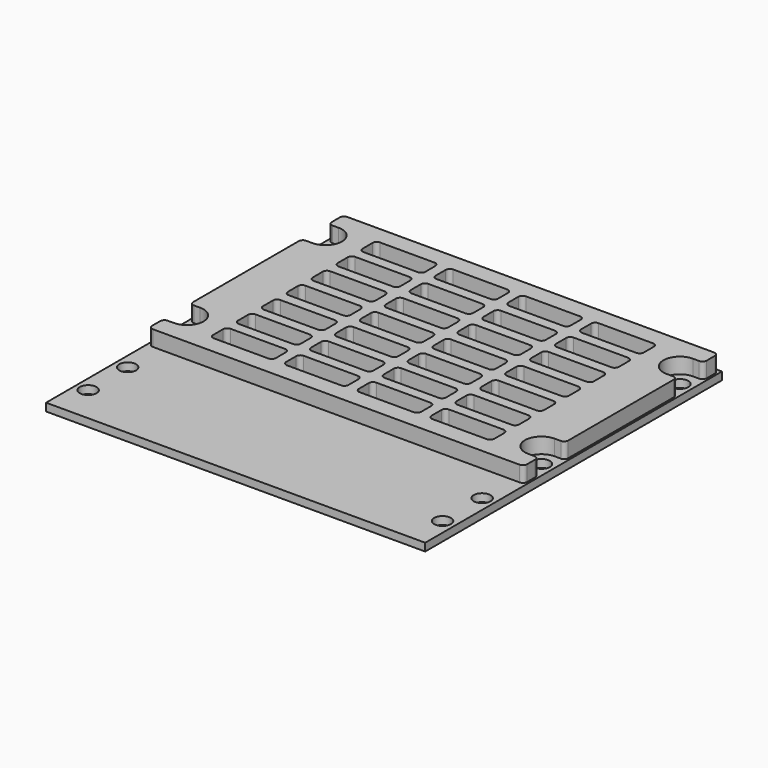
from build123d import *

# Parameters (mm, degrees)
F0_R      = 3.24
F1_DEPTH  = 3
F2_DEPTH  = 6
F3_R      = 1.588
F4_W      = 24
F4_H      = 8
F4_W_2    = 24.1504099965
F5_DEPTH  = 25
F6_R      = 1.588
F6_2_R    = 1.588
F7_W      = 108.300819993
F7_H      = 80
F8_DEPTH  = 25
F9_R      = 3.24
F10_DEPTH = 3


# Not quite as in the source:
# - a feature names something its author has since deleted; it is built from what else it names


with BuildPart() as f1:
    # F0 (on Top) → F1 (new body)
    with BuildSketch(Plane.XY):
        Polygon((0, 57.15), (-73.025, 57.15), (-73.025, 9.525), (-73.025, -38.1), (73.025, -38.1), (73.025, 57.15), align=None)
        with Locations((-68.262, -23.812)):
            Circle(F0_R, mode=Mode.SUBTRACT)
        with Locations((68.262, -23.812)):
            Circle(F0_R, mode=Mode.SUBTRACT)
        with Locations((-68.262, 42.862)):
            Circle(F0_R, mode=Mode.SUBTRACT)
        with BuildLine():
            Line((-72.225, -17.461), (-72.225, 9.525))
            Line((-72.225, 9.525), (-72.225, 36.511))
            Line((-72.225, 36.511), (-68.262, 36.511))
            ThreePointArc((-68.262, 36.511), (-61.911, 42.862), (-68.262, 49.213))
            Line((-68.262, 49.213), (-72.225, 49.213))
            Line((-72.225, 49.213), (-72.225, 56.35))
            Line((-72.225, 56.35), (72.225, 56.35))
            Line((72.225, 56.35), (72.225, 49.213))
            Line((72.225, 49.213), (68.262, 49.213))
            ThreePointArc((68.262, 49.213), (61.911, 42.862), (68.262, 36.511))
            Line((68.262, 36.511), (72.225, 36.511))
            Line((72.225, 36.511), (72.225, -17.461))
            Line((72.225, -17.461), (68.262, -17.461))
            ThreePointArc((68.262, -17.461), (61.911, -23.812), (68.262, -30.163))
            Line((68.262, -30.163), (72.225, -30.163))
            Line((72.225, -30.163), (72.225, -37.3))
            Line((72.225, -37.3), (-72.225, -37.3))
            Line((-72.225, -37.3), (-72.225, -30.163))
            Line((-72.225, -30.163), (-68.262, -30.163))
            ThreePointArc((-68.262, -30.163), (-61.911, -23.812), (-68.262, -17.461))
            Line((-68.262, -17.461), (-72.225, -17.461))
        make_face(mode=Mode.SUBTRACT)
        with Locations((68.262, 42.862)):
            Circle(F0_R, mode=Mode.SUBTRACT)
        with BuildLine():
            Line((-72.225, 36.511), (-72.225, 9.525))
            Line((-72.225, 9.525), (-72.225, -17.461))
            Line((-72.225, -17.461), (-68.262, -17.461))
            ThreePointArc((-68.262, -17.461), (-61.911, -23.812), (-68.262, -30.163))
            Line((-68.262, -30.163), (-72.225, -30.163))
            Line((-72.225, -30.163), (-72.225, -37.3))
            Line((-72.225, -37.3), (72.225, -37.3))
            Line((72.225, -37.3), (72.225, -30.163))
            Line((72.225, -30.163), (68.262, -30.163))
            ThreePointArc((68.262, -30.163), (61.911, -23.812), (68.262, -17.461))
            Line((68.262, -17.461), (72.225, -17.461))
            Line((72.225, -17.461), (72.225, 36.511))
            Line((72.225, 36.511), (68.262, 36.511))
            ThreePointArc((68.262, 36.511), (61.911, 42.862), (68.262, 49.213))
            Line((68.262, 49.213), (72.225, 49.213))
            Line((72.225, 49.213), (72.225, 56.35))
            Line((72.225, 56.35), (-72.225, 56.35))
            Line((-72.225, 56.35), (-72.225, 49.213))
            Line((-72.225, 49.213), (-68.262, 49.213))
            ThreePointArc((-68.262, 49.213), (-61.911, 42.862), (-68.262, 36.511))
            Line((-68.262, 36.511), (-72.225, 36.511))
        make_face()
    extrude(amount=-F1_DEPTH)


with BuildPart() as f2:
    # F0 (on Top) → F2 (new body)
    with BuildSketch(Plane.XY):
        with BuildLine():
            Line((-72.225, 36.511), (-72.225, 9.525))
            Line((-72.225, 9.525), (-72.225, -17.461))
            Line((-72.225, -17.461), (-68.262, -17.461))
            ThreePointArc((-68.262, -17.461), (-61.911, -23.812), (-68.262, -30.163))
            Line((-68.262, -30.163), (-72.225, -30.163))
            Line((-72.225, -30.163), (-72.225, -37.3))
            Line((-72.225, -37.3), (72.225, -37.3))
            Line((72.225, -37.3), (72.225, -30.163))
            Line((72.225, -30.163), (68.262, -30.163))
            ThreePointArc((68.262, -30.163), (61.911, -23.812), (68.262, -17.461))
            Line((68.262, -17.461), (72.225, -17.461))
            Line((72.225, -17.461), (72.225, 36.511))
            Line((72.225, 36.511), (68.262, 36.511))
            ThreePointArc((68.262, 36.511), (61.911, 42.862), (68.262, 49.213))
            Line((68.262, 49.213), (72.225, 49.213))
            Line((72.225, 49.213), (72.225, 56.35))
            Line((72.225, 56.35), (-72.225, 56.35))
            Line((-72.225, 56.35), (-72.225, 49.213))
            Line((-72.225, 49.213), (-68.262, 49.213))
            ThreePointArc((-68.262, 49.213), (-61.911, 42.862), (-68.262, 36.511))
            Line((-68.262, 36.511), (-72.225, 36.511))
        make_face()
    extrude(amount=F2_DEPTH)

    # F3
    f3_edges = [f2.edges().sort_by_distance(p)[0] for p in [
        (-72.225, 56.35, 3),
        (-72.225, -37.3, 3),
        (72.225, -37.3, 3),
        (72.225, 56.35, 3),
        (-72.225, 36.511, 3),
        (-72.225, -17.461, 3),
        (-72.225, 49.213, 3),
        (72.225, 49.213, 3),
        (72.225, 36.511, 3),
        (72.225, -17.461, 3),
        (72.225, -30.163, 3),
        (-72.225, -30.163, 3),
    ]]
    fillet(f3_edges, radius=F3_R)


with BuildPart() as f5_tool:
    # F4 (on face) → F5 (new body)
    with BuildSketch(Plane.XY.offset(6)):
        with Locations((-14, 45.525)):
            Rectangle(F4_W, F4_H)
        with Locations((-42.0752049983, 45.525)):
            Rectangle(F4_W_2, F4_H)
        with Locations((42.0752049983, 45.525)):
            Rectangle(F4_W_2, F4_H)
        with Locations((14, 45.525)):
            Rectangle(F4_W, F4_H)
        with Locations((-14, 33.525)):
            Rectangle(F4_W, F4_H)
        with Locations((-42.0752049983, 33.525)):
            Rectangle(F4_W_2, F4_H)
        with Locations((14, 33.525)):
            Rectangle(F4_W, F4_H)
        with Locations((42.0752049983, 33.525)):
            Rectangle(F4_W_2, F4_H)
        with Locations((-14, 21.525)):
            Rectangle(F4_W, F4_H)
        with Locations((-42.0752049983, 21.525)):
            Rectangle(F4_W_2, F4_H)
        with Locations((14, 21.525)):
            Rectangle(F4_W, F4_H)
        with Locations((42.0752049983, 21.525)):
            Rectangle(F4_W_2, F4_H)
        Polygon((-2, 9.525), (-2, 13.525), (-26, 13.525), (-26, 5.525), (-2, 5.525), align=None)
        with Locations((-42.0752049983, 9.525)):
            Rectangle(F4_W_2, F4_H)
        with Locations((14, 9.525)):
            Rectangle(F4_W, F4_H)
        with Locations((42.0752049983, 9.525)):
            Rectangle(F4_W_2, F4_H)
        with Locations((-14, -2.475)):
            Rectangle(F4_W, F4_H)
        with Locations((-42.0752049983, -2.475)):
            Rectangle(F4_W_2, F4_H)
        with Locations((14, -2.475)):
            Rectangle(F4_W, F4_H)
        with Locations((42.0752049983, -2.475)):
            Rectangle(F4_W_2, F4_H)
        with Locations((-14, -14.475)):
            Rectangle(F4_W, F4_H)
        with Locations((-42.0752049983, -14.475)):
            Rectangle(F4_W_2, F4_H)
        with Locations((14, -14.475)):
            Rectangle(F4_W, F4_H)
        with Locations((42.0752049983, -14.475)):
            Rectangle(F4_W_2, F4_H)
        with Locations((-14, -26.475)):
            Rectangle(F4_W, F4_H)
        with Locations((-42.0752049983, -26.475)):
            Rectangle(F4_W_2, F4_H)
        with Locations((14, -26.475)):
            Rectangle(F4_W, F4_H)
        with Locations((42.0752049983, -26.475)):
            Rectangle(F4_W_2, F4_H)
    extrude(amount=-F5_DEPTH)


with BuildPart() as f1_1:
    add(f1.part)

    # F5: cut by f5_tool
    add(f5_tool.part, mode=Mode.SUBTRACT)

    # F6
    f6_edges = [f1_1.edges().sort_by_distance(p)[0] for p in [
        (-30, 41.525, -1.5),
        (-30, 37.525, -1.5),
        (-30, 25.525, -1.5),
        (-30, 13.525, -1.5),
        (-30, 1.525, -1.5),
        (-30, -10.475, -1.5),
        (-30, -22.475, -1.5),
        (-2, -22.475, -1.5),
        (-2, -10.475, -1.5),
        (-2, 1.525, -1.5),
        (-2, 13.525, -1.5),
        (-2, 25.525, -1.5),
        (-2, 37.525, -1.5),
        (26, 37.525, -1.5),
        (26, 25.525, -1.5),
        (26, 13.525, -1.5),
        (26, 1.525, -1.5),
        (26, -10.475, -1.5),
        (26, -22.475, -1.5),
        (-2, 41.525, -1.5),
        (26, 41.525, -1.5),
        (-30, 29.525, -1.5),
        (-2, 29.525, -1.5),
        (26, 29.525, -1.5),
        (26, 17.525, -1.5),
        (-2, 17.525, -1.5),
        (-30, 17.525, -1.5),
        (-30, 5.525, -1.5),
        (-30, -6.475, -1.5),
        (-30, -18.475, -1.5),
        (-2, -18.475, -1.5),
        (-2, -6.475, -1.5),
        (-2, 5.525, -1.5),
        (26, 5.525, -1.5),
        (26, -6.475, -1.5),
        (26, -18.475, -1.5),
        (-26, 41.525, -1.5),
        (2, 41.525, -1.5),
        (30, 41.525, -1.5),
        (30, 29.525, -1.5),
        (2, 29.525, -1.5),
        (-26, 29.525, -1.5),
        (-26, 17.525, -1.5),
        (2, 17.525, -1.5),
        (30, 17.525, -1.5),
        (30, 5.525, -1.5),
        (2, 5.525, -1.5),
        (-26, 5.525, -1.5),
        (-26, -6.475, -1.5),
        (2, -6.475, -1.5),
        (30, -6.475, -1.5),
        (30, -18.475, -1.5),
        (2, -18.475, -1.5),
        (-26, -18.475, -1.5),
        (-26, 37.525, -1.5),
        (2, 37.525, -1.5),
        (30, 37.525, -1.5),
        (-26, 25.525, -1.5),
        (2, 25.525, -1.5),
        (30, 25.525, -1.5),
        (-26, 13.525, -1.5),
        (2, 13.525, -1.5),
        (30, 13.525, -1.5),
        (-26, 1.525, -1.5),
        (2, 1.525, -1.5),
        (30, 1.525, -1.5),
        (-26, -10.475, -1.5),
        (2, -10.475, -1.5),
        (30, -10.475, -1.5),
        (-26, -22.475, -1.5),
        (2, -22.475, -1.5),
        (30, -22.475, -1.5),
    ]]
    fillet(f6_edges, radius=F6_R)

    # F7 (on face) → F8 (cut)
    with BuildSketch(Plane(origin=(0, 0, -3), x_dir=(1, 0, 0), z_dir=(0, 0, -1))):
        with Locations((0, -9.525)):
            Rectangle(F7_W, F7_H)
    extrude(amount=-F8_DEPTH, mode=Mode.SUBTRACT)

    # F9 (on face) → F10 (join)
    with BuildSketch(Plane(origin=(0, 0, -3), x_dir=(1, 0, 0), z_dir=(0, 0, -1))):
        Polygon((-73.025, 61.9125), (-73.025, 38.1), (73.025, 38.1), (73.025, 85.725), (-73.025, 85.725), align=None)
        with Locations((-68.262, 52.388)):
            Circle(F9_R, mode=Mode.SUBTRACT)
        with Locations((68.262, 52.388)):
            Circle(F9_R, mode=Mode.SUBTRACT)
        with Locations((-68.262, 71.437)):
            Circle(F9_R, mode=Mode.SUBTRACT)
        with Locations((68.262, 71.437)):
            Circle(F9_R, mode=Mode.SUBTRACT)
    extrude(amount=-F10_DEPTH)


with BuildPart() as f2_1:
    add(f2.part)

    # F5: cut by f5_tool
    add(f5_tool.part, mode=Mode.SUBTRACT)

    # F6#2
    f6_2_edges = [f2_1.edges().sort_by_distance(p)[0] for p in [
        (-54.15041, 49.525, 3),
        (-54.15041, 41.525, 3),
        (-30, 41.525, 3),
        (-30, 49.525, 3),
        (-30, 37.525, 3),
        (-30, 25.525, 3),
        (-30, 13.525, 3),
        (-30, 1.525, 3),
        (-30, -10.475, 3),
        (-30, -22.475, 3),
        (-2, -22.475, 3),
        (-2, -10.475, 3),
        (-2, 1.525, 3),
        (-2, 13.525, 3),
        (-2, 25.525, 3),
        (-2, 37.525, 3),
        (-2, 49.525, 3),
        (26, 49.525, 3),
        (26, 37.525, 3),
        (26, 25.525, 3),
        (26, 13.525, 3),
        (26, 1.525, 3),
        (26, -10.475, 3),
        (26, -22.475, 3),
        (54.15041, -22.475, 3),
        (54.15041, -10.475, 3),
        (54.15041, 1.525, 3),
        (54.15041, 13.525, 3),
        (54.15041, 25.525, 3),
        (54.15041, 37.525, 3),
        (54.15041, 49.525, 3),
        (-2, 41.525, 3),
        (26, 41.525, 3),
        (54.15041, 41.525, 3),
        (-30, 29.525, 3),
        (-2, 29.525, 3),
        (26, 29.525, 3),
        (54.15041, 29.525, 3),
        (54.15041, 17.525, 3),
        (26, 17.525, 3),
        (-2, 17.525, 3),
        (-30, 17.525, 3),
        (-30, 5.525, 3),
        (-30, -6.475, 3),
        (-30, -18.475, 3),
        (-30, -30.475, 3),
        (-2, -30.475, 3),
        (-2, -18.475, 3),
        (-2, -6.475, 3),
        (-2, 5.525, 3),
        (26, 5.525, 3),
        (54.15041, 5.525, 3),
        (26, -6.475, 3),
        (54.15041, -6.475, 3),
        (54.15041, -18.475, 3),
        (26, -18.475, 3),
        (26, -30.475, 3),
        (54.15041, -30.475, 3),
        (-26, 41.525, 3),
        (2, 41.525, 3),
        (30, 41.525, 3),
        (30, 29.525, 3),
        (2, 29.525, 3),
        (-26, 29.525, 3),
        (-54.15041, 29.525, 3),
        (-54.15041, 17.525, 3),
        (-26, 17.525, 3),
        (2, 17.525, 3),
        (30, 17.525, 3),
        (30, 5.525, 3),
        (2, 5.525, 3),
        (-26, 5.525, 3),
        (-54.15041, 5.525, 3),
        (-54.15041, -6.475, 3),
        (-26, -6.475, 3),
        (2, -6.475, 3),
        (30, -6.475, 3),
        (30, -18.475, 3),
        (2, -18.475, 3),
        (-26, -18.475, 3),
        (-54.15041, -18.475, 3),
        (-54.15041, -30.475, 3),
        (-26, -30.475, 3),
        (2, -30.475, 3),
        (30, -30.475, 3),
        (-26, 49.525, 3),
        (2, 49.525, 3),
        (30, 49.525, 3),
        (-54.15041, 37.525, 3),
        (-26, 37.525, 3),
        (2, 37.525, 3),
        (30, 37.525, 3),
        (-54.15041, 25.525, 3),
        (-26, 25.525, 3),
        (2, 25.525, 3),
        (30, 25.525, 3),
        (-54.15041, 13.525, 3),
        (-26, 13.525, 3),
        (2, 13.525, 3),
        (30, 13.525, 3),
        (-54.15041, 1.525, 3),
        (-26, 1.525, 3),
        (2, 1.525, 3),
        (30, 1.525, 3),
        (-54.15041, -10.475, 3),
        (-26, -10.475, 3),
        (2, -10.475, 3),
        (30, -10.475, 3),
        (-54.15041, -22.475, 3),
        (-26, -22.475, 3),
        (2, -22.475, 3),
        (30, -22.475, 3),
    ]]
    fillet(f6_2_edges, radius=F6_2_R)


solid = Compound([f1_1.part, f2_1.part])
